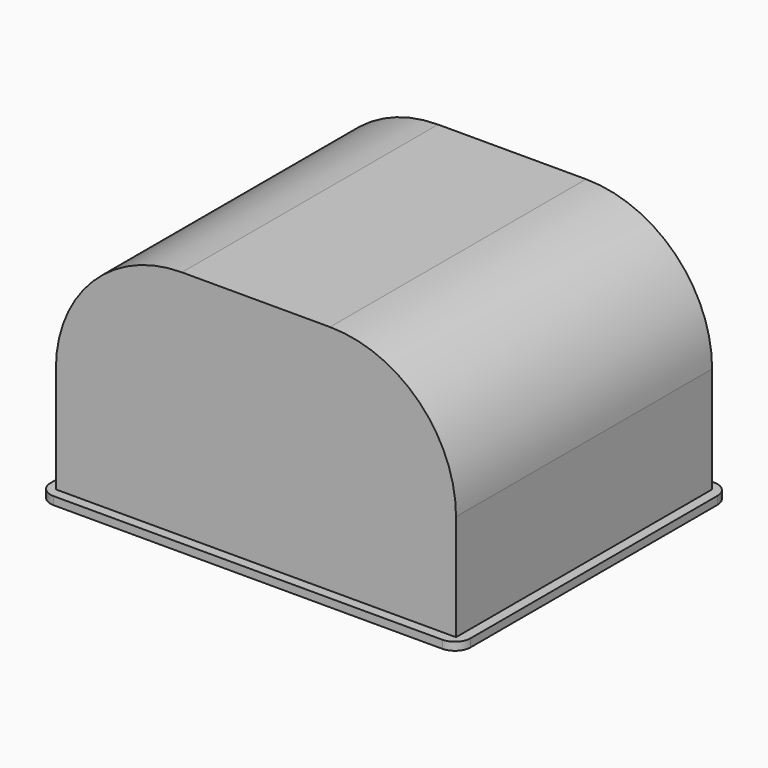
from build123d import *

# Parameters (mm, degrees)
F0_W     = 133.35
F0_H     = 107.95
F1_DEPTH = 76.2
F2_W     = 127
F2_H     = 101.6
F3_DEPTH = 76.2
F4_DEPTH = 73.66
F5_DEPTH = 76.2
F6_T     = -2.5
F7_R     = 40
F8_R     = 4
F9_R     = 5
F10_R    = 40


with BuildPart() as f1:
    # F0 (on Top) → F1 (new body)
    with BuildSketch(Plane.XY):
        Rectangle(F0_W, F0_H)
    extrude(amount=F1_DEPTH)

    # F2 (on Top) → F3 (cut)
    with BuildSketch(Plane.XY):
        Rectangle(F2_W, F2_H)
    extrude(amount=F3_DEPTH, mode=Mode.SUBTRACT)

    # F4 (cut): a face of the model
    f4_faces = [f1.faces().sort_by_distance(p)[0] for p in [
        (64.9593244771, 0, 76.2),
    ]]
    extrude(f4_faces, amount=-F4_DEPTH, mode=Mode.SUBTRACT)

    # F2 (on Top) → F5 (join)
    with BuildSketch(Plane.XY):
        Rectangle(F2_W, F2_H)
    extrude(amount=F5_DEPTH)

    # F6
    f6_openings = [f1.faces().sort_by_distance(p)[0] for p in [
        (0, 0, 0),
    ]]
    offset(amount=F6_T, openings=f6_openings, kind=Kind.INTERSECTION)

    # F7
    f7_edges = [f1.edges().sort_by_distance(p)[0] for p in [
        (-61, 0, 73.7),
        (61, 0, 73.7),
    ]]
    fillet(f7_edges, radius=F7_R)

    # F8
    f8_edges = [f1.edges().sort_by_distance(p)[0] for p in [
        (-49.284271, -48.3, 61.984271),
        (49.284271, 48.3, 61.984271),
    ]]
    fillet(f8_edges, radius=F8_R)

    # F9
    f9_edges = [f1.edges().sort_by_distance(p)[0] for p in [
        (66.675, 53.975, 1.27),
        (66.675, -53.975, 1.27),
        (-66.675, -53.975, 1.27),
        (-66.675, 53.975, 1.27),
    ]]
    fillet(f9_edges, radius=F9_R)

    # F10
    f10_edges = [f1.edges().sort_by_distance(p)[0] for p in [
        (-63.5, 0, 76.2),
        (63.5, 0, 76.2),
    ]]
    fillet(f10_edges, radius=F10_R)


solid = f1.part
